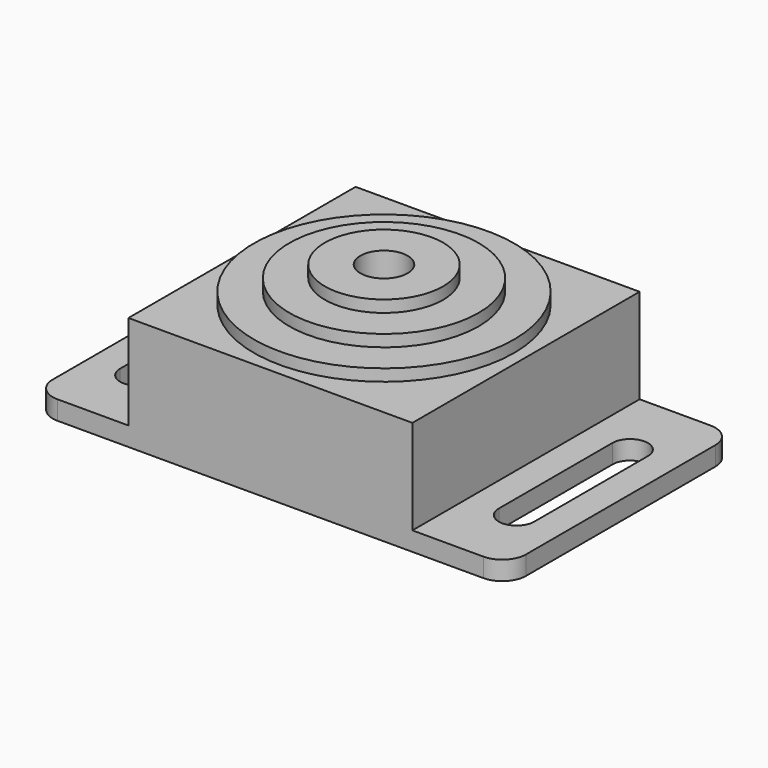
from build123d import *

# Parameters (mm, degrees)
F0_W      = 127
F0_H      = 76.2
F1_DEPTH  = 5.08
F2_W      = 76.2
F2_H      = 76.2
F3_DEPTH  = 25.4
F4_R      = 28.575
F5_DEPTH  = 25.4
F6_R      = 6.35
F8_DEPTH  = 25.4
F9_R      = 34.925
F10_DEPTH = 3.175
F11_R     = 27.6225
F12_DEPTH = 25.146
F13_R     = 19.05
F14_DEPTH = 31.496
F15_R     = 9.525
F16_DEPTH = 5.08
F17_R     = 25.4
F18_DEPTH = 3.175
F19_R     = 19.05
F20_DEPTH = 28.448
F21_R     = 12.7
F22_DEPTH = 31.623
F23_R     = 15.875
F24_DEPTH = 3.175
F25_R     = 9.525
F26_DEPTH = 31.496
F27_R     = 6.35
F28_DEPTH = 30.48
F29_R     = 3.175
F30_DEPTH = 25.4


# Not quite as in the source:
# - a pattern or mirror of a feature is missing from the dataset's text; its kind, count and spacing are read off the source's solid


with BuildPart() as f1:
    # F0 (on Top) → F1 (new body)
    with BuildSketch(Plane.XY):
        Rectangle(F0_W, F0_H)
    extrude(amount=F1_DEPTH)

    # F2 (on face) → F3 (join)
    with BuildSketch(Plane.XY.offset(5.08)):
        Rectangle(F2_W, F2_H)
    extrude(amount=F3_DEPTH)

    # F4 (on face) → F5 (cut)
    with BuildSketch(Plane.XY.offset(30.48)):
        Circle(F4_R)
    extrude(amount=-F5_DEPTH, mode=Mode.SUBTRACT)

    # F6
    f6_edges = [f1.edges().sort_by_distance(p)[0] for p in [
        (63.5, -38.1, 2.54),
        (63.5, 38.1, 2.54),
        (-63.5, 38.1, 2.54),
        (-63.5, -38.1, 2.54),
    ]]
    fillet(f6_edges, radius=F6_R)

    # F7 (on face) → F8 (cut)
    with BuildSketch(Plane.XY.offset(5.08)):
        with BuildLine():
            Line((-46.0375, -19.05), (-46.0375, 19.05))
            ThreePointArc((-46.0375, 19.05), (-50.8, 23.8125), (-55.5625, 19.05))
            Line((-55.5625, 19.05), (-55.5625, -19.05))
            ThreePointArc((-55.5625, -19.05), (-50.8, -23.8125), (-46.0375, -19.05))
        make_face()
    f8 = extrude(amount=-F8_DEPTH, mode=Mode.SUBTRACT)

    # F8_copies: F8 across plane
    add(f8.mirror(Plane(origin=(0, 0, 0), x_dir=(0, 0, 1), z_dir=(1, 0, 0))), mode=Mode.SUBTRACT)

    # F15 (on face) → F16 (cut, through all)
    with BuildSketch(Plane(origin=(0, 0, 0), x_dir=(1, 0, 0), z_dir=(0, 0, -1))):
        Circle(F15_R)
    extrude(amount=-F16_DEPTH, mode=Mode.SUBTRACT)


with BuildPart() as f10:
    # F9 (on face) → F10 (new body)
    with BuildSketch(Plane.XY.offset(30.48)):
        Circle(F9_R)
    extrude(amount=F10_DEPTH)

    # F11 (on face) → F12 (join)
    with BuildSketch(Plane.XY.offset(30.48)):
        Circle(F11_R)
    extrude(amount=-F12_DEPTH)

    # F13 (on face) → F14 (cut)
    with BuildSketch(Plane.XY.offset(33.655)):
        Circle(F13_R)
    extrude(amount=-F14_DEPTH, mode=Mode.SUBTRACT)


with BuildPart() as f18:
    # F17 (on face) → F18 (new body)
    with BuildSketch(Plane.XY.offset(33.655)):
        Circle(F17_R)
    extrude(amount=F18_DEPTH)

    # F19 (on face) → F20 (join)
    with BuildSketch(Plane(origin=(0, 0, 33.655), x_dir=(1, 0, 0), z_dir=(0, 0, -1))):
        Circle(F19_R)
    extrude(amount=F20_DEPTH)

    # F21 (on face) → F22 (cut, through all)
    with BuildSketch(Plane.XY.offset(36.83)):
        Circle(F21_R)
    extrude(amount=-F22_DEPTH, mode=Mode.SUBTRACT)


with BuildPart() as f24:
    # F23 (on face) → F24 (new body)
    with BuildSketch(Plane.XY.offset(36.83)):
        Circle(F23_R)
    extrude(amount=F24_DEPTH)

    # F25 (on face) → F26 (join)
    with BuildSketch(Plane(origin=(0, 0, 36.83), x_dir=(1, 0, 0), z_dir=(0, 0, -1))):
        Circle(F25_R)
    extrude(amount=F26_DEPTH)

    # F27 (on face) → F28 (cut)
    with BuildSketch(Plane.XY.offset(40.005)):
        Circle(F27_R)
    extrude(amount=-F28_DEPTH, mode=Mode.SUBTRACT)

    # F29 (on face) → F30 (cut)
    with BuildSketch(Plane(origin=(0, 0, 5.334), x_dir=(1, 0, 0), z_dir=(0, 0, -1))):
        Circle(F29_R)
    extrude(amount=-F30_DEPTH, mode=Mode.SUBTRACT)


solid = Compound([f1.part, f10.part, f18.part, f24.part])
